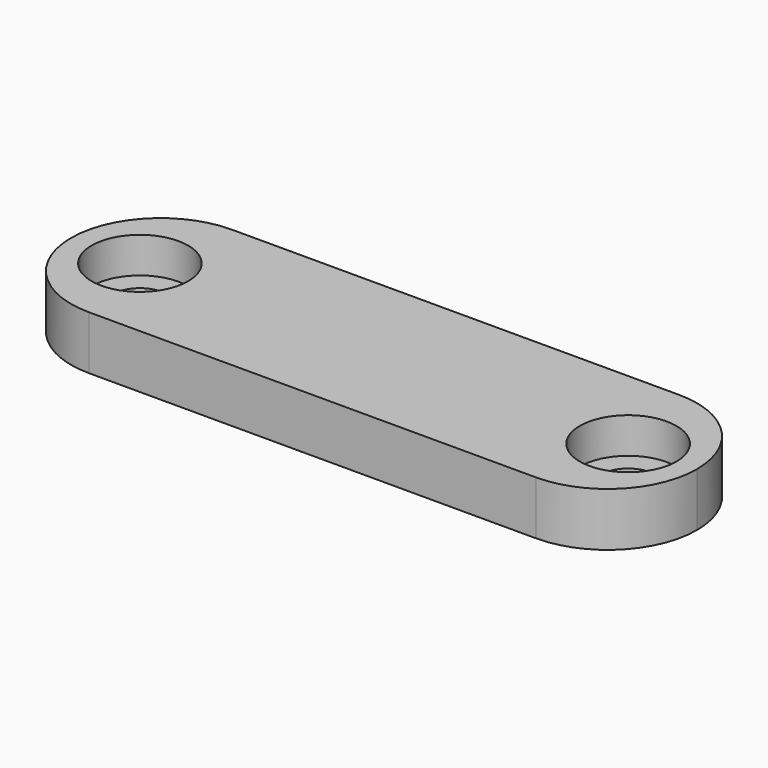
from build123d import *

# Parameters (mm, degrees)
F0_W           = 35
F0_H           = 10
F0_W_2         = 20
F0_H_2         = 5
F1_DEPTH       = 3
F4_D           = 3
F4_CBORE_D     = 5.4
F4_CBORE_DEPTH = 2
F5_R           = 4.99999


# Not quite as in the source:
# - a fillet or chamfer is up to 0.001 mm smaller than in the source, because OpenCascade refuses the exact size


with BuildPart() as f1:
    # F0 (on Top) → F1 (new body)
    with BuildSketch(Plane.XY):
        Rectangle(F0_W, F0_H)
        Rectangle(F0_W_2, F0_H_2, mode=Mode.SUBTRACT)
        Rectangle(F0_W_2, F0_H_2)
    extrude(amount=F1_DEPTH)

    # F4 (through all)
    with Locations(Plane.XY.offset(3)):
        with Locations((-13.65, 0), (13.65, 0)):
            CounterBoreHole(F4_D / 2, F4_CBORE_D / 2, F4_CBORE_DEPTH)

    # F5 (radius 5 in the source; OpenCascade refuses exactly that, so slightly less here)
    f5_edges = [f1.edges().sort_by_distance(p)[0] for p in [
        (-17.5, -5, 1.5),
        (-17.5, 5, 1.5),
        (17.5, 5, 1.5),
        (17.5, -5, 1.5),
    ]]
    fillet(f5_edges, radius=F5_R)


solid = f1.part
